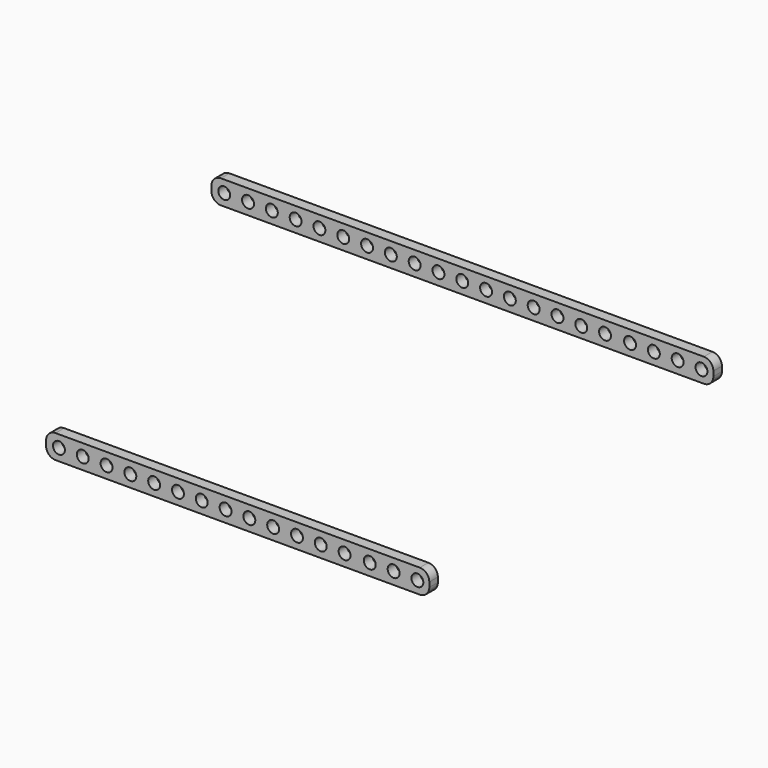
from build123d import *

# Parameters (mm, degrees)
F0_R     = 2.5
F1_DEPTH = 4.5
F2_DEPTH = 4.5


# Not quite as in the source:
# - a feature names something its author has since deleted; it is built from what else it names


with BuildPart() as f1:
    # F0 (on Front) → F1 (new body)
    with BuildSketch(Plane.XZ):
        with BuildLine():
            Line((173.4446543215, 22.8161337823), (-29.448286426, 22.8161337823))
            ThreePointArc((-29.448286426, 22.8161337823), (-32.2767135507, 21.6445609071), (-33.448286426, 18.8161337823))
            Line((-33.448286426, 18.8161337823), (-33.448286426, 16.8161337823))
            ThreePointArc((-33.448286426, 16.8161337823), (-32.2767135507, 13.9877066576), (-29.448286426, 12.8161337823))
            Line((-29.448286426, 12.8161337823), (173.4446543215, 12.8161337823))
            ThreePointArc((173.4446543215, 12.8161337823), (176.2730814463, 13.9877066576), (177.4446543215, 16.8161337823))
            Line((177.4446543215, 16.8161337823), (177.4446543215, 18.8161337823))
            ThreePointArc((177.4446543215, 18.8161337823), (176.2730814463, 21.6445609071), (173.4446543215, 22.8161337823))
        make_face()
        with Locations((-28.048286426, 17.8161337823)):
            Circle(F0_R, mode=Mode.SUBTRACT)
        with Locations((-18.048286426, 17.8161337823)):
            Circle(F0_R, mode=Mode.SUBTRACT)
        with Locations((-8.048286426, 17.8161337823)):
            Circle(F0_R, mode=Mode.SUBTRACT)
        with Locations((1.951713574, 17.8161337823)):
            Circle(F0_R, mode=Mode.SUBTRACT)
        with Locations((11.951713574, 17.8161337823)):
            Circle(F0_R, mode=Mode.SUBTRACT)
        with Locations((21.951713574, 17.8161337823)):
            Circle(F0_R, mode=Mode.SUBTRACT)
        with Locations((31.951713574, 17.8161337823)):
            Circle(F0_R, mode=Mode.SUBTRACT)
        with Locations((41.951713574, 17.8161337823)):
            Circle(F0_R, mode=Mode.SUBTRACT)
        with Locations((51.951713574, 17.8161337823)):
            Circle(F0_R, mode=Mode.SUBTRACT)
        with Locations((61.951713574, 17.8161337823)):
            Circle(F0_R, mode=Mode.SUBTRACT)
        with Locations((71.951713574, 17.8161337823)):
            Circle(F0_R, mode=Mode.SUBTRACT)
        with Locations((81.951713574, 17.8161337823)):
            Circle(F0_R, mode=Mode.SUBTRACT)
        with Locations((91.951713574, 17.8161337823)):
            Circle(F0_R, mode=Mode.SUBTRACT)
        with Locations((101.951713574, 17.8161337823)):
            Circle(F0_R, mode=Mode.SUBTRACT)
        with Locations((111.951713574, 17.8161337823)):
            Circle(F0_R, mode=Mode.SUBTRACT)
        with Locations((121.951713574, 17.4404541092)):
            Circle(F0_R, mode=Mode.SUBTRACT)
        with Locations((131.9446543215, 17.8161337823)):
            Circle(F0_R, mode=Mode.SUBTRACT)
        with Locations((142.4452806723, 17.8161337823)):
            Circle(F0_R, mode=Mode.SUBTRACT)
        with Locations((152.4452806723, 17.8161337823)):
            Circle(F0_R, mode=Mode.SUBTRACT)
        with Locations((162.4452806723, 17.9280561807)):
            Circle(F0_R, mode=Mode.SUBTRACT)
        with Locations((172.4446543215, 17.8161337823)):
            Circle(F0_R, mode=Mode.SUBTRACT)
    extrude(amount=F1_DEPTH)


with BuildPart() as f2:
    # F0 (on Front) → F2 (new body)
    with BuildSketch(Plane.XZ):
        with BuildLine():
            Line((54.1081197957, -94.0042481228), (-98.8918802043, -94.0042481228))
            ThreePointArc((-98.8918802043, -94.0042481228), (-101.720307329, -95.175820998), (-102.8918802043, -98.0042481228))
            Line((-102.8918802043, -98.0042481228), (-102.8918802043, -100.0042481228))
            ThreePointArc((-102.8918802043, -100.0042481228), (-101.720307329, -102.8326752475), (-98.8918802043, -104.0042481228))
            Line((-98.8918802043, -104.0042481228), (54.1081197957, -104.0042481228))
            ThreePointArc((54.1081197957, -104.0042481228), (56.9365469205, -102.8326752475), (58.1081197957, -100.0042481228))
            Line((58.1081197957, -100.0042481228), (58.1081197957, -98.0042481228))
            ThreePointArc((58.1081197957, -98.0042481228), (56.9365469205, -95.175820998), (54.1081197957, -94.0042481228))
        make_face()
        with Locations((-97.4918802043, -99.0042481228)):
            Circle(F0_R, mode=Mode.SUBTRACT)
        with Locations((-87.4918802043, -99.0042481228)):
            Circle(F0_R, mode=Mode.SUBTRACT)
        with Locations((-77.4918802043, -99.0042481228)):
            Circle(F0_R, mode=Mode.SUBTRACT)
        with Locations((-67.4918802043, -99.0042481228)):
            Circle(F0_R, mode=Mode.SUBTRACT)
        with Locations((-57.4918802043, -99.0042481228)):
            Circle(F0_R, mode=Mode.SUBTRACT)
        with Locations((-47.4918802043, -99.0042481228)):
            Circle(F0_R, mode=Mode.SUBTRACT)
        with Locations((-37.4918802043, -99.0042481228)):
            Circle(F0_R, mode=Mode.SUBTRACT)
        with Locations((-27.4918802043, -99.0042481228)):
            Circle(F0_R, mode=Mode.SUBTRACT)
        with Locations((-17.4918802043, -99.0042481228)):
            Circle(F0_R, mode=Mode.SUBTRACT)
        with Locations((-7.4918802043, -99.0042481228)):
            Circle(F0_R, mode=Mode.SUBTRACT)
        with Locations((2.5081197957, -99.0042481228)):
            Circle(F0_R, mode=Mode.SUBTRACT)
        with Locations((12.5081197957, -99.0042481228)):
            Circle(F0_R, mode=Mode.SUBTRACT)
        with Locations((22.5081197957, -99.0042481228)):
            Circle(F0_R, mode=Mode.SUBTRACT)
        with Locations((33.1087461465, -99.0042481228)):
            Circle(F0_R, mode=Mode.SUBTRACT)
        with Locations((43.1087461465, -98.8923257244)):
            Circle(F0_R, mode=Mode.SUBTRACT)
        with Locations((53.1081197957, -99.0042481228)):
            Circle(F0_R, mode=Mode.SUBTRACT)
    extrude(amount=F2_DEPTH)


solid = Compound([f1.part, f2.part])
